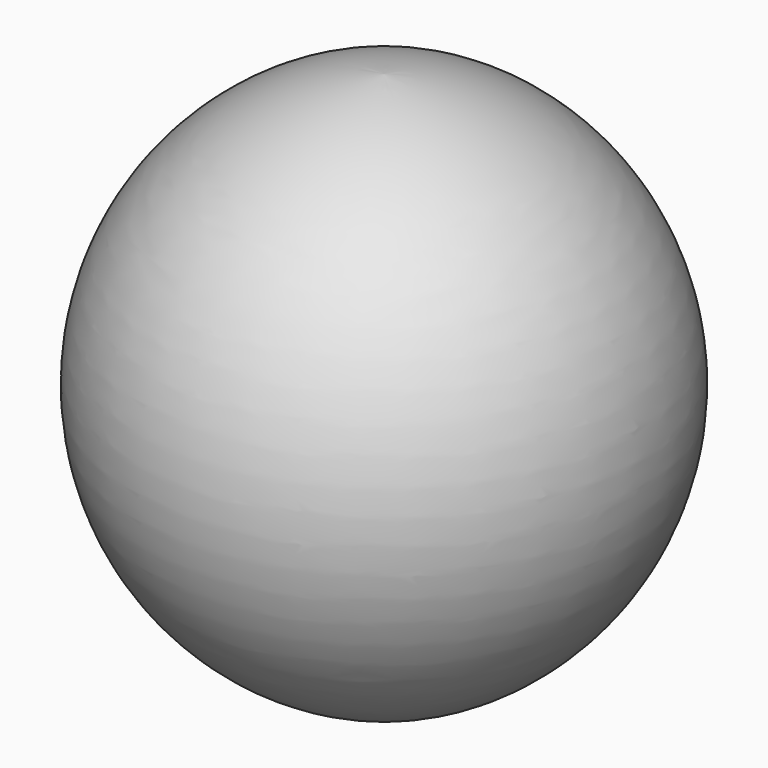
from build123d import *


# Not quite as in the source:
# - a feature of the source that left no trace in its solid (it failed there, or was rolled back) is left out


with BuildPart() as f1:
    # F0 (on Front) → F1 (revolve)
    with BuildSketch(Plane.XZ):
        with BuildLine():
            Line((0, -53.2572120428), (0, 52.9885739088))
            ThreePointArc((0, 52.9885739088), (-49.110734819, -0.134319067), (0, -53.2572120428))
        make_face()
    revolve(axis=Axis((0, 0, -0.134319067), (0, 0, -1)))


solid = f1.part
